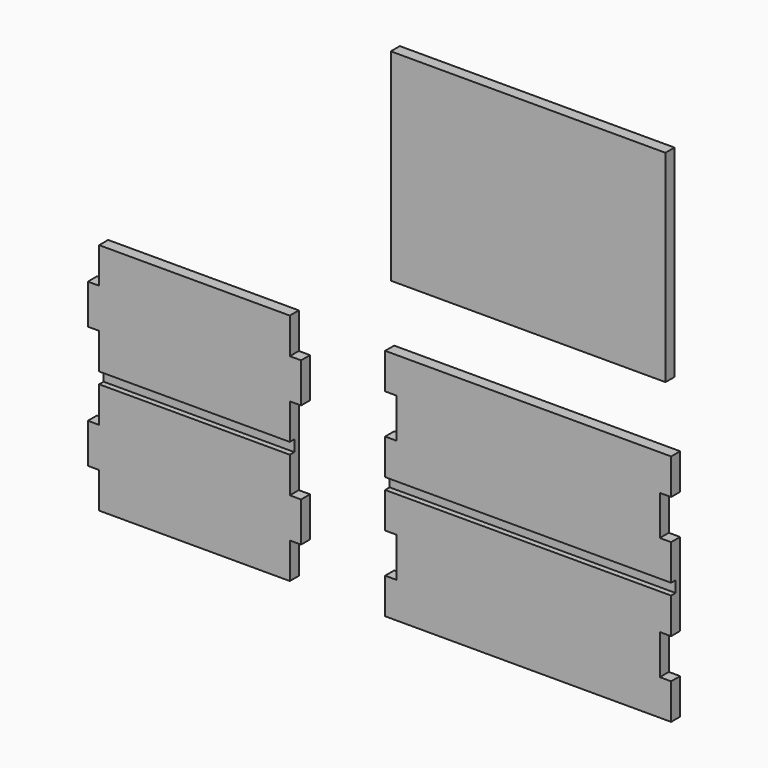
from build123d import *

# Parameters (mm, degrees)
F1_W     = 18.034
F1_H     = 63.5
F2_DEPTH = 18.034
F1_W_2   = 439.166
F1_H_2   = 322.834
F1_W_3   = 304.8
F1_H_3   = 18.034
F3_DEPTH = 9.017
F1_W_4   = 457.2


# Not quite as in the source:
# - a variable given as a bare number and used for a length is read in inches; the dataset says mm whatever the document's units were
# - a feature names something its author has since deleted; it is built from what else it names


with BuildPart() as f2:
    # F1 (on Front) → F2 (new body)
    with BuildSketch(Plane.XZ):
        Polygon((-381, 129.667), (-381, 186.817), (-685.8, 186.817), (-685.8, 129.667), (-685.8, 66.167), (-685.8, 9.017), (-381, 9.017), (-381, 66.167), align=None)
        with Locations((-694.817, 97.917)):
            Rectangle(F1_W, F1_H)
        with Locations((-371.983, 97.917)):
            Rectangle(F1_W, F1_H)
    extrude(amount=F2_DEPTH)



with BuildPart() as f2b:
    # F1 (on Front) → F2, piece 2 (new body)
    with BuildSketch(Plane.XZ):
        with Locations((-694.817, -97.917)):
            Rectangle(F1_W, F1_H)
        with Locations((-371.983, -97.917)):
            Rectangle(F1_W, F1_H)
        Polygon((-381, -66.167), (-381, -9.017), (-685.8, -9.017), (-685.8, -66.167), (-685.8, -129.667), (-685.8, -186.817), (-381, -186.817), (-381, -129.667), align=None)
    extrude(amount=F2_DEPTH)


with BuildPart() as f2c:
    # F1 (on Front) → F2, piece 3 (new body)
    with BuildSketch(Plane.XZ):
        Polygon((228.6, -9.017), (-228.6, -9.017), (-228.6, -66.167), (-210.566, -66.167), (-210.566, -129.667), (-228.6, -129.667), (-228.6, -186.817), (228.6, -186.817), (228.6, -129.667), (210.566, -129.667), (210.566, -66.167), (228.6, -66.167), align=None)
    extrude(amount=F2_DEPTH)



with BuildPart() as f2d:
    # F1 (on Front) → F2, piece 4 (new body)
    with BuildSketch(Plane.XZ):
        Polygon((228.6, 186.817), (-228.6, 186.817), (-228.6, 129.667), (-210.566, 129.667), (-210.566, 66.167), (-228.6, 66.167), (-228.6, 9.017), (228.6, 9.017), (228.6, 66.167), (210.566, 66.167), (210.566, 129.667), (228.6, 129.667), align=None)
    extrude(amount=F2_DEPTH)


with BuildPart() as f2e:
    # F1 (on Front) → F2, piece 5 (new body)
    with BuildSketch(Plane.XZ):
        with Locations((0, 449.834)):
            Rectangle(F1_W_2, F1_H_2)
    extrude(amount=F2_DEPTH)


with BuildPart() as f2_1:
    add(f2.part)

    add(f2b.part)  # F3 merges F2b
    # F1 (on Front) → F3 (join)
    with BuildSketch(Plane.XZ):
        with Locations((-533.4, 0)):
            Rectangle(F1_W_3, F1_H_3)
    extrude(amount=F3_DEPTH)


with BuildPart() as f2c_1:
    add(f2c.part)

    add(f2d.part)  # F3#2 merges F2d
    # F1 (on Front) → F3, piece 2 (join)
    with BuildSketch(Plane.XZ):
        Rectangle(F1_W_4, F1_H_3)
    extrude(amount=F3_DEPTH)


solid = Compound([f2e.part, f2_1.part, f2c_1.part])
